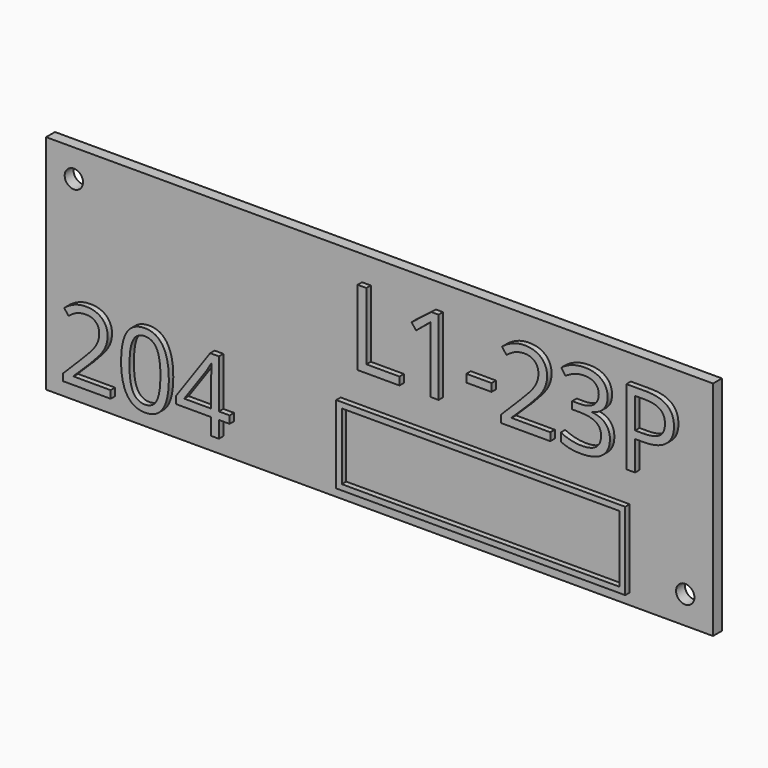
from build123d import *

# Parameters (mm, degrees)
F0_W         = 120
F0_H         = 40
F1_DEPTH     = 2
F3_D         = 3.3
F4_TEXT_SIZE = 18.9181200118
F5_DEPTH     = 1
F6_TEXT_SIZE = 18.1818181818
F7_DEPTH     = 1
F8_W         = 52
F8_H         = 14
F8_W_2       = 49.99999962
F8_H_2       = 11.99999962
F9_DEPTH     = 1


# Not quite as in the source:
# - Text() gives the source's letters only with a copy of the font that has no kerning and outlines rounded to 1/6400 em; it was checked with that copy


with BuildPart() as f1:
    # F0 (on Front) → F1 (new body)
    with BuildSketch(Plane.XZ):
        Rectangle(F0_W, F0_H)
    extrude(amount=F1_DEPTH)

    # F3 (through all)
    with Locations(Plane.XZ.offset(2)):
        with Locations((-55, 15), (55, -15)):
            Hole(F3_D / 2)

    # F4 (on face) → F5 (join)
    with BuildSketch(Plane.XZ.offset(2)):
        with Locations((-5, 2)):
            Text('L1-23P', F4_TEXT_SIZE, font='Open Sans', text_align=(TextAlign.LEFT, TextAlign.BOTTOM))
    extrude(amount=F5_DEPTH)

    # F6 (on face) → F7 (join)
    with BuildSketch(Plane.XZ.offset(2)):
        with Locations((-57, -17)):
            Text('204', F6_TEXT_SIZE, font='Open Sans', text_align=(TextAlign.LEFT, TextAlign.BOTTOM))
    extrude(amount=F7_DEPTH)

    # F8 (on face) → F9 (join)
    with BuildSketch(Plane.XZ.offset(2)):
        with Locations((19, -11)):
            Rectangle(F8_W, F8_H)
        with Locations((19, -11)):
            Rectangle(F8_W_2, F8_H_2, mode=Mode.SUBTRACT)
    extrude(amount=F9_DEPTH)


solid = f1.part
